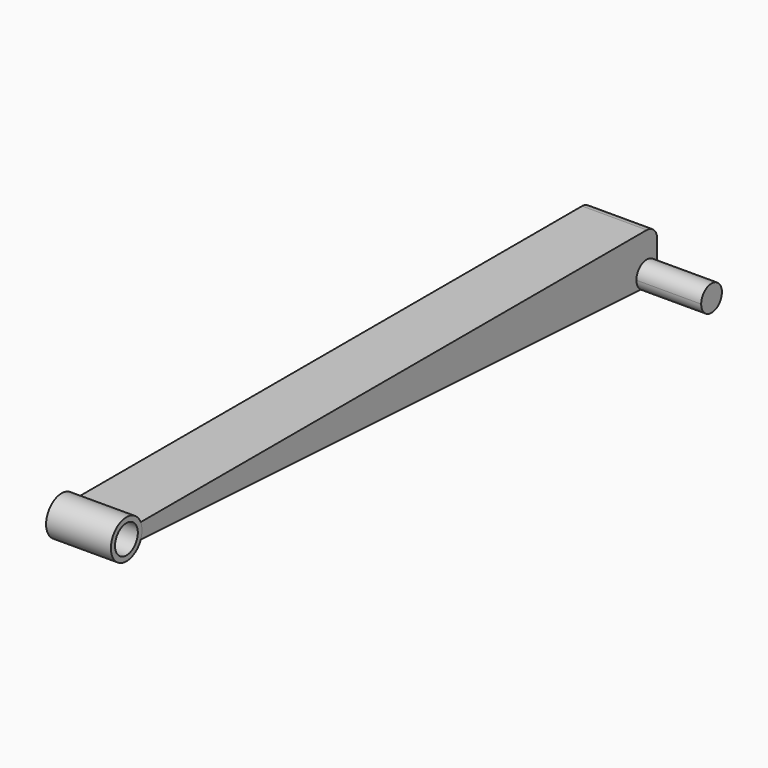
from build123d import *

# Parameters (mm, degrees)
F0_R      = 7.5
F0_R_2    = 5.5
F1_DEPTH  = 25
F3_W      = 24.975579232
F3_H      = 6
F4_DEPTH  = 250
F5_W      = 10
F5_H      = 20
F6_DEPTH  = 24.975579232
F7_R      = 5
F8_R      = 4.99999
F10_DEPTH = 25
F12_DEPTH = 24.975579232


# Not quite as in the source:
# - a fillet or chamfer is up to 0.001 mm smaller than in the source, because OpenCascade refuses the exact size


with BuildPart() as f1:
    # F0 (on Right) → F1 (new body)
    with BuildSketch(Plane.YZ):
        Circle(F0_R)
        Circle(F0_R_2, mode=Mode.SUBTRACT)
    extrude(amount=F1_DEPTH)

    # F3 (on offset) → F4 (join)
    with BuildSketch(Plane.XZ.offset(-6)):
        with Locations((12.487789616, 0)):
            Rectangle(F3_W, F3_H)
    extrude(amount=-F4_DEPTH)

    # F5 (on face) → F6 (join, through all)
    with BuildSketch(Plane.YZ.offset(24.975579232)):
        with Locations((251, -7)):
            Rectangle(F5_W, F5_H)
    extrude(amount=-F6_DEPTH)

    # F7
    f7_edges = [f1.edges().sort_by_distance(p)[0] for p in [
        (12.48779, 256, 3),
        (12.48779, 246, -3),
    ]]
    fillet(f7_edges, radius=F7_R)

    # F8 (radius 5 in the source; OpenCascade refuses exactly that, so slightly less here)
    f8_edges = [f1.edges().sort_by_distance(p)[0] for p in [
        (12.48779, 246, -17),
        (12.48779, 256, -17),
    ]]
    fillet(f8_edges, radius=F8_R)

    # F9 (on face) → F10 (join)
    with BuildSketch(Plane.YZ.offset(24.975579232)):
        with BuildLine():
            ThreePointArc((256, -12), (251, -7), (246, -12))
            ThreePointArc((246, -12), (247.4644660941, -15.5355339059), (251, -17))
            ThreePointArc((251, -17), (254.5355339059, -15.5355339059), (256, -12))
        make_face()
    extrude(amount=F10_DEPTH)

    # F11 (on face) → F12 (join, through all)
    with BuildSketch(Plane.YZ.offset(24.975579232)):
        Polygon((6.8738635424, -3), (248.2517808676, -16.0908978432), (251, -6.9958104675), (6.8738635424, 3), align=None)
    extrude(amount=-F12_DEPTH)


solid = f1.part
